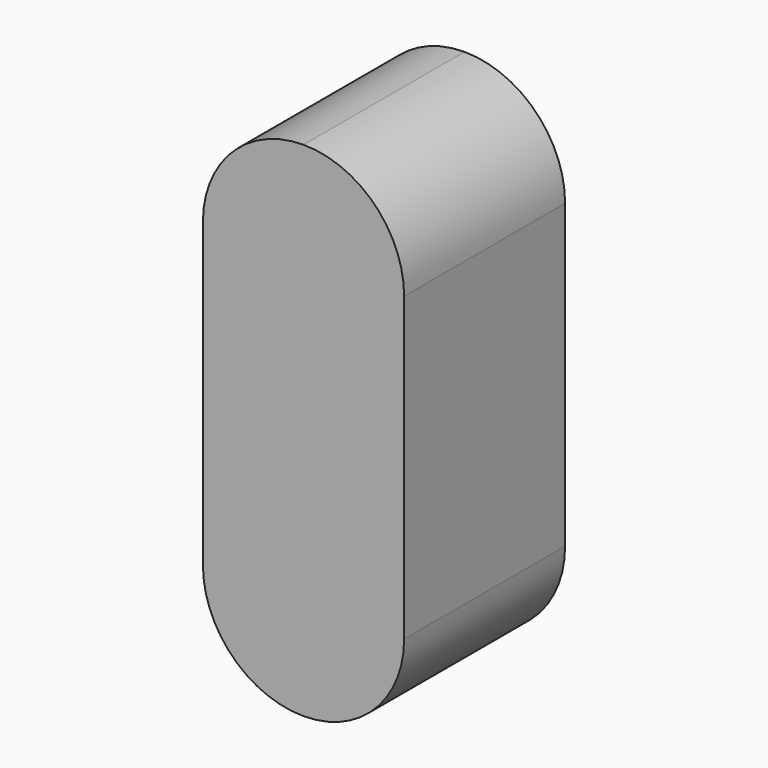
from build123d import *

# Parameters (mm, degrees)
F0_W     = 4
F0_H     = 10
F1_DEPTH = 4
F2_R     = 1.99999


# Not quite as in the source:
# - a fillet or chamfer is up to 0.001 mm smaller than in the source, because OpenCascade refuses the exact size


with BuildPart() as f1:
    # F0 (on Front) → F1 (new body)
    with BuildSketch(Plane.XZ):
        Rectangle(F0_W, F0_H)
    extrude(amount=F1_DEPTH)

    # F2 (radius 2 in the source; OpenCascade refuses exactly that, so slightly less here)
    f2_edges = [f1.edges().sort_by_distance(p)[0] for p in [
        (2, -2, 5),
        (2, -2, -5),
        (-2, -2, 5),
        (-2, -2, -5),
    ]]
    fillet(f2_edges, radius=F2_R)


solid = f1.part
